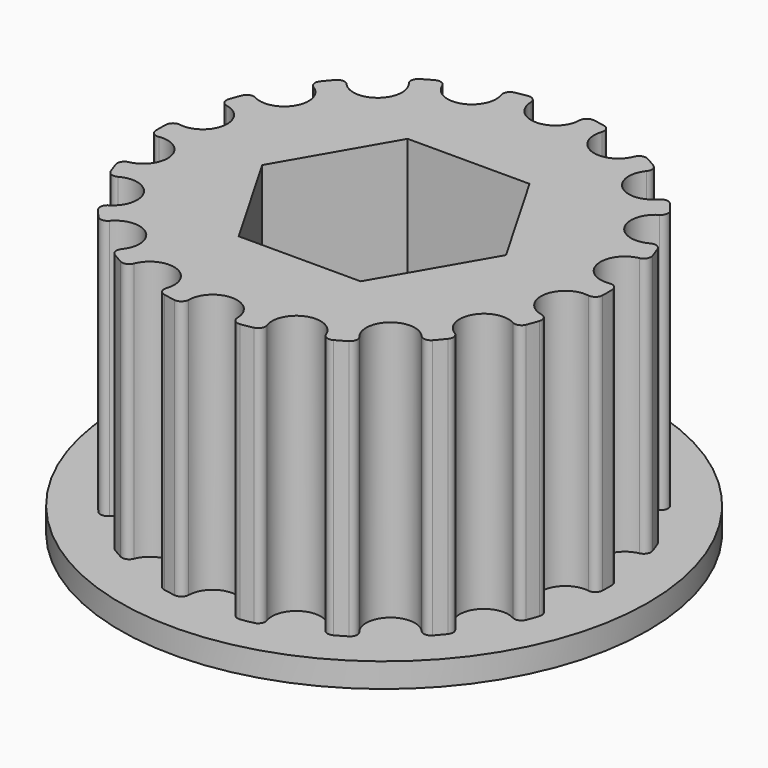
from build123d import *

# Parameters (mm, degrees)
F2_R            = 13.7514448946
F3_DEPTH        = 16
F5_DEPTH        = 16
F5_COPIES_COUNT = 18
F8_R            = 16.2514448946
F8_R_2          = 13.7514448946
F9_DEPTH        = 1.5
F10_DEPTH       = 17.501


# Not quite as in the source:
# - a feature of the source that left no trace in its solid (it failed there, or was rolled back) is left out
# - a pattern or mirror of a feature is missing from the dataset's text; its kind, count and spacing are read off the source's solid


with BuildPart() as f3:
    # F2 (on Top) → F3 (new body)
    with BuildSketch(Plane.XY):
        Circle(F2_R)
    extrude(amount=F3_DEPTH)

    # F4 (on face) → F5 (cut, through all)
    with BuildSketch(Plane.XY.offset(16)):
        with BuildLine():
            ThreePointArc((-2.015669756, 13.6029155744), (-1.6587079327, 13.5010225766), (-1.499776395, 13.1655457628))
            ThreePointArc((-1.499776395, 13.1655457628), (0, 11.6914448946), (1.499776395, 13.1655457628))
            ThreePointArc((1.499776395, 13.1655457628), (1.6587079327, 13.5010225766), (2.015669756, 13.6029155744))
            ThreePointArc((2.015669756, 13.6029155744), (0, 13.7514448946), (-2.015669756, 13.6029155744))
        make_face()
    f5 = extrude(amount=-F5_DEPTH, mode=Mode.SUBTRACT)

    # F5_copies: F5 ×18 about axis
    f5_copies_axis = Axis((0, 0, 0), (0, 0, 1))
    for i in range(1, F5_COPIES_COUNT):
        add(f5.rotate(f5_copies_axis, i * 360 / F5_COPIES_COUNT), mode=Mode.SUBTRACT)

    # F8 (on face) + F2 (on Top) → F9 (join)
    with BuildSketch(Plane.XY):
        Circle(F8_R)
        Circle(F8_R_2, mode=Mode.SUBTRACT)
    with BuildSketch(Plane.XY):
        Circle(F2_R)
    extrude(amount=-F9_DEPTH)

    # F7 (on face) → F10 (cut, through all)
    with BuildSketch(Plane.XY.offset(16)):
        Polygon((3.7527767497, 6.5), (-3.7527767497, 6.5), (-7.5055534995, 0), (-3.7527767497, -6.5), (3.7527767497, -6.5), (7.5055534995, 0), align=None)
    extrude(amount=-F10_DEPTH, mode=Mode.SUBTRACT)


solid = f3.part
